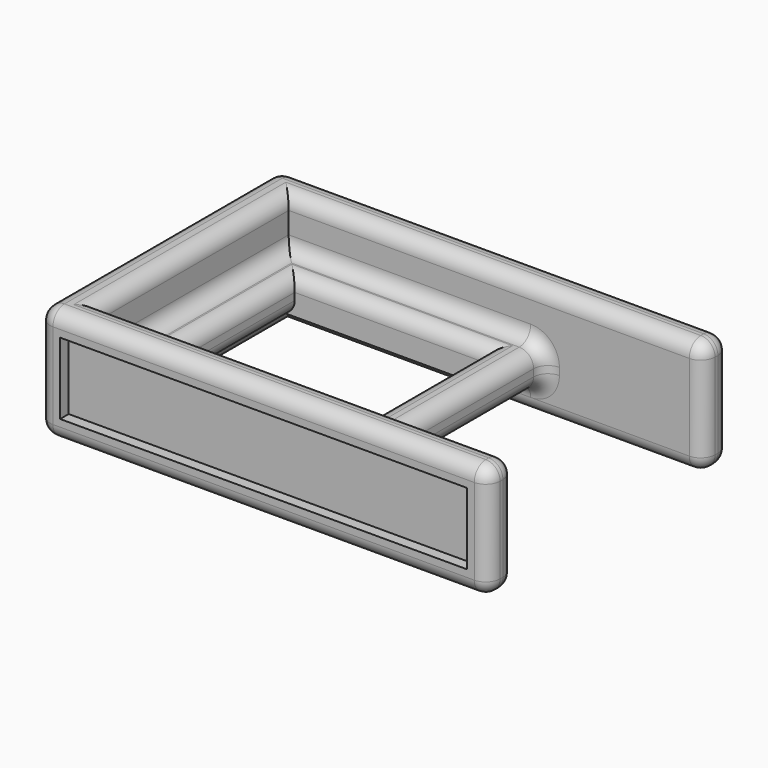
from build123d import *

# Parameters (mm, degrees)
F0_W      = 33.4
F0_H      = 23
F1_DEPTH  = 8
F0_W_2    = 17.8890476892
F0_H_2    = 16.5
F2_DEPTH  = 4.5
F3_DEPTH  = 1
F4_DEPTH  = 1
F5_DEPTH  = 1
F6_DEPTH  = 1
F7_DEPTH  = 2
F8_W      = 13.3992488682
F8_H      = 12.2999999374
F9_DEPTH  = 3.4
F11_W     = 28.4
F11_H     = 5
F12_DEPTH = 0.75
F13_W     = 28.4
F13_H     = 5
F14_DEPTH = 0.75
F15_W     = 18
F15_H     = 5
F16_DEPTH = 1.75
F10_W     = 16.5
F10_H     = 8
F17_DEPTH = 2.5
F18_R     = 0.99999


# Not quite as in the source:
# - a fillet or chamfer is up to 0.001 mm smaller than in the source, because OpenCascade refuses the exact size
# - a feature names something its author has since deleted; it is built from what else it names


with BuildPart() as f1:
    # F0 (on Top) → F1 (new body)
    with BuildSketch(Plane.XY):
        with Locations((-3.299, -0.375)):
            Rectangle(F0_W, F0_H)
        Polygon((1.3400476892, 7.875), (9.951, 7.875), (9.951, -8.625), (1.3400476892, -8.625), (-16.549, -8.625), (-16.549, 7.875), align=None, mode=Mode.SUBTRACT)
    extrude(amount=F1_DEPTH)

    # F0 (on Top) → F2 (join)
    with BuildSketch(Plane.XY):
        with Locations((-7.6044761554, -0.375)):
            Rectangle(F0_W_2, F0_H_2)
    extrude(amount=F2_DEPTH)

    # F3 (cut): a face of the model
    f3_faces = [f1.faces().sort_by_distance(p)[0] for p in [
        (-3.299, -11.875, 4),
    ]]
    extrude(f3_faces, amount=-F3_DEPTH, mode=Mode.SUBTRACT)

    # F4 (cut): a face of the model
    f4_faces = [f1.faces().sort_by_distance(p)[0] for p in [
        (13.401, 0.125, 4),
    ]]
    extrude(f4_faces, amount=-F4_DEPTH, mode=Mode.SUBTRACT)

    # F5 (cut): a face of the model
    f5_faces = [f1.faces().sort_by_distance(p)[0] for p in [
        (-3.799, 11.125, 4),
    ]]
    extrude(f5_faces, amount=-F5_DEPTH, mode=Mode.SUBTRACT)

    # F6 (cut): a face of the model
    f6_faces = [f1.faces().sort_by_distance(p)[0] for p in [
        (-19.999, -0.375, 4),
    ]]
    extrude(f6_faces, amount=-F6_DEPTH, mode=Mode.SUBTRACT)

    # F0 (on Top) → F7 (cut)
    with BuildSketch(Plane.XY):
        with Locations((-7.6044761554, -0.375)):
            Rectangle(F0_W_2, F0_H_2)
    extrude(amount=F7_DEPTH, mode=Mode.SUBTRACT)

    # F8 (on face) → F9 (cut)
    with BuildSketch(Plane(origin=(0, 0, 2), x_dir=(1, 0, 0), z_dir=(0, 0, -1))):
        with Locations((-7.7493755346, 0.375)):
            Rectangle(F8_W, F8_H)
    extrude(amount=-F9_DEPTH, mode=Mode.SUBTRACT)

    # F11 (on face) → F12 (cut)
    with BuildSketch(Plane.XZ.offset(10.875)):
        with Locations((-3.299, 4)):
            Rectangle(F11_W, F11_H)
    extrude(amount=-F12_DEPTH, mode=Mode.SUBTRACT)

    # F13 (on face) → F14 (cut)
    with BuildSketch(Plane(origin=(0, 10.125, 0), x_dir=(-1, 0, 0), z_dir=(0, 1, 0))):
        with Locations((3.299, 4)):
            Rectangle(F13_W, F13_H)
    extrude(amount=-F14_DEPTH, mode=Mode.SUBTRACT)

    # F15 (on face) → F16 (cut)
    with BuildSketch(Plane(origin=(-18.999, 0, 0), x_dir=(0, -1, 0), z_dir=(-1, 0, 0))):
        with Locations((0.375, 4)):
            Rectangle(F15_W, F15_H)
    extrude(amount=-F16_DEPTH, mode=Mode.SUBTRACT)

    # F10 (on face) → F17 (cut)
    with BuildSketch(Plane.YZ.offset(12.401)):
        with Locations((-0.375, 4)):
            Rectangle(F10_W, F10_H)
    extrude(amount=-F17_DEPTH, mode=Mode.SUBTRACT)

    # F18 (radius 1 in the source; OpenCascade refuses exactly that, so slightly less here)
    f18_edges = [f1.edges().sort_by_distance(p)[0] for p in [
        (-3.299, 10.125, 8),
        (-2.074, 7.875, 8),
        (-18.999, -0.375, 8),
        (-16.549, -0.375, 8),
        (-2.074, -8.625, 8),
        (-3.299, -10.875, 8),
        (12.401, -9.75, 8),
        (12.401, 9, 8),
        (12.401, 9, 0),
        (12.401, -9.75, 0),
        (-3.299, 10.125, 0),
        (-3.299, -10.875, 0),
        (-18.999, -0.375, 0),
        (-2.074, -8.625, 0),
        (-16.549, -0.375, 0),
        (-2.074, 7.875, 0),
        (12.401, -10.875, 4),
        (12.401, -8.625, 4),
        (12.401, 7.875, 4),
        (12.401, 10.125, 4),
        (-18.999, -10.875, 4),
        (-18.999, 10.125, 4),
        (-14.449, -0.375, 4.5),
        (-1.049751, -0.375, 4.5),
        (-7.604476, 7.875, 2),
        (-16.549, -0.375, 2),
        (-7.604476, -8.625, 2),
        (-1.049751, -0.375, 2),
        (-14.449, -0.375, 2),
        (-16.549, -0.375, 4.5),
        (1.340048, -0.375, 4.5),
        (1.340048, -0.375, 2),
        (1.340048, 7.875, 3.25),
        (-7.604476, 7.875, 4.5),
        (-7.604476, -8.625, 4.5),
        (-7.749376, -6.525, 4.5),
        (-7.749376, 5.775, 4.5),
        (1.340048, -8.625, 3.25),
    ]]
    fillet(f18_edges, radius=F18_R)


solid = f1.part
